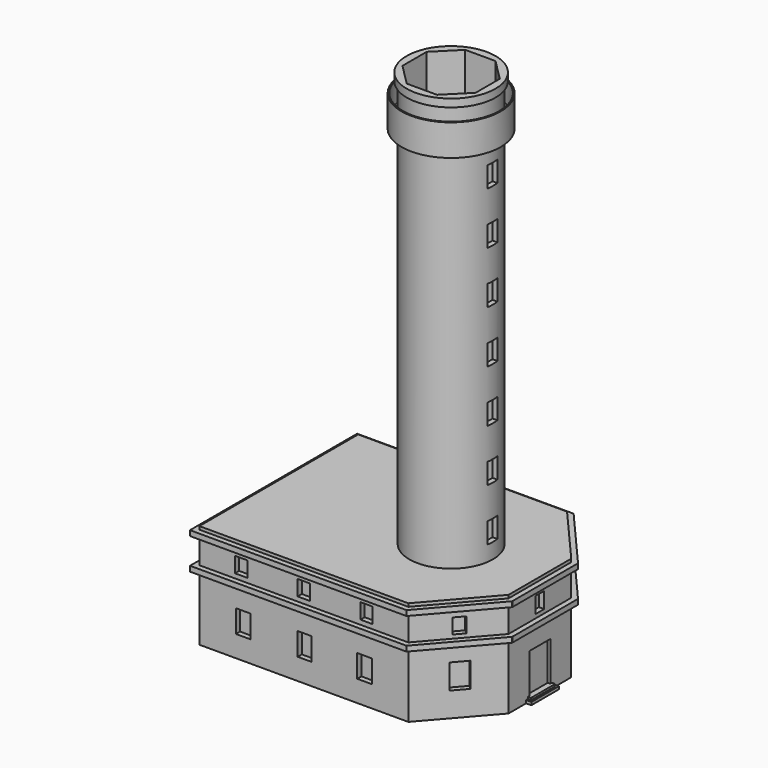
from build123d import *

# Parameters (mm, degrees)
F1_DEPTH  = 50.8
F2_R      = 20.32
F3_DEPTH  = 177.8
F5_DEPTH  = 381
F6_W      = 101.6
F6_H      = 2.54
F7_DEPTH  = 2.54
F8_W      = 38.7089666615
F8_H      = 2.54
F9_DEPTH  = 2.54
F10_DEPTH = 1.143
F11_DEPTH = 1.143
F12_DEPTH = 1.143
F13_DEPTH = 1.143
F14_W     = 38.1
F14_H     = 2.54
F15_DEPTH = 2.54
F16_DEPTH = 0.889
F17_DEPTH = 0.889
F18_W     = 38.7089666615
F18_H     = 2.54
F19_DEPTH = 2.54
F20_W     = 101.6
F20_H     = 2.54
F21_DEPTH = 2.54
F22_DEPTH = 0.889
F23_DEPTH = 0.889
F24_DEPTH = 1.143
F25_DEPTH = 1.143
F27_DEPTH = 2.54
F29_DEPTH = 1.27
F30_DEPTH = 1.524
F31_DEPTH = 2.54
F28_W     = 5.0940667279
F28_H     = 7.758654654
F32_DEPTH = 2.54
F33_R     = 24.13
F33_R_2   = 20.32
F34_DEPTH = 5.08
F35_R     = 20.32
F36_DEPTH = 15.24
F37_R     = 21.59
F37_R_2   = 20.32
F38_DEPTH = 3.81
F39_R     = 24.13
F39_R_2   = 23.495
F40_DEPTH = 10.16
F41_W     = 6.827371195
F41_H     = 9.7158756107
F41_W_2   = 11.0288318247
F41_H_2   = 20.7330156118
F41_W_3   = 6.8273767829
F41_H_3   = 8.1403255463
F41_W_4   = 6.0395970941
F42_DEPTH = 2.54
F43_W     = 7.0659834892
F43_H     = 11.040600948
F43_W_2   = 6.8451717962
F43_W_3   = 5.9624109417
F43_H_2   = 7.5072459877
F43_W_4   = 5.9624111746
F44_DEPTH = 2.54
F45_W     = 9.3363560736
F45_H     = 11.9140176103
F45_W_2   = 5.0487220287
F45_H_2   = 6.8554915488
F46_DEPTH = 2.54
F47_W     = 8.1120701507
F47_H     = 12.0682595298
F47_W_2   = 5.420149304
F47_H_2   = 7.3144324124
F48_DEPTH = 2.54
F49_W     = 5.7560801506
F49_H     = 7.2415210307
F49_W_2   = 8.1699229777
F49_H_2   = 11.5121612325
F49_W_3   = 10.0267203525
F49_H_3   = 19.1327799112
F50_DEPTH = 2.54
F51_W     = 5.8573530426
F51_H     = 10.0520360901
F52_DEPTH = 25.4
F53_W     = 5.1205269992
F53_H     = 8.2716196775
F54_DEPTH = 15.24


with BuildPart() as f1:
    # F0 (on Top) → F1 (new body)
    with BuildSketch(Plane.XY):
        Polygon((-50.8, -48.26), (50.8, -48.26), (76.2, -19.05), (76.2, 19.05), (50.8, 48.26), (-50.8, 48.26), align=None)
    extrude(amount=F1_DEPTH)

    # F2 (on face) → F3 (join)
    with BuildSketch(Plane.XY.offset(50.8)):
        with Locations((33.02, 0)):
            Circle(F2_R)
    extrude(amount=F3_DEPTH)

    # F4 (on Top) → F5 (cut)
    with BuildSketch(Plane.XY):
        Polygon((50.8, 0), (50.8, 7.364717139), (40.384717139, 17.78), (25.655282861, 17.78), (15.24, 7.364717139), (15.24, -7.364717139), (25.655282861, -17.78), (40.384717139, -17.78), (50.8, -7.364717139), align=None)
    extrude(amount=F5_DEPTH, mode=Mode.SUBTRACT)

    # F6 (on face) → F7 (join)
    with BuildSketch(Plane(origin=(0, 48.26, 0), x_dir=(-1, 0, 0), z_dir=(0, 1, 0))):
        with Locations((0, 48.006)):
            Rectangle(F6_W, F6_H)
        with Locations((0, 32.766)):
            Rectangle(F6_W, F6_H)
    extrude(amount=F7_DEPTH)

    # F8 (on face) → F9 (join)
    with BuildSketch(Plane(origin=(52.8232508073, 45.9332615716, 0), x_dir=(-0.6561787149, 0.7546055222, 0), z_dir=(0.7546055222, 0.6561787149, 0))):
        with Locations((-16.2710995493, 48.006)):
            Rectangle(F8_W, F8_H)
        with Locations((-16.2710995493, 32.766)):
            Rectangle(F8_W, F8_H)
    extrude(amount=F9_DEPTH)

    # F10 (add): a face of the model
    f10_faces = [f1.faces().sort_by_distance(p)[0] for p in [
        (50.8, 49.53, 48.006),
    ]]
    extrude(f10_faces, amount=F10_DEPTH)

    # F11 (add): a face of the model
    f11_faces = [f1.faces().sort_by_distance(p)[0] for p in [
        (52.3298490131, 49.5903034897, 48.006),
    ]]
    extrude(f11_faces, amount=F11_DEPTH)

    # F12 (add): a face of the model
    f12_faces = [f1.faces().sort_by_distance(p)[0] for p in [
        (50.8, 49.53, 32.766),
    ]]
    extrude(f12_faces, amount=F12_DEPTH)

    # F13 (add): a face of the model
    f13_faces = [f1.faces().sort_by_distance(p)[0] for p in [
        (52.3298490131, 49.5903034897, 32.766),
    ]]
    extrude(f13_faces, amount=F13_DEPTH)

    # F14 (on face) → F15 (join)
    with BuildSketch(Plane.YZ.offset(76.2)):
        with Locations((0, 48.006)):
            Rectangle(F14_W, F14_H)
        with Locations((0, 32.766)):
            Rectangle(F14_W, F14_H)
    extrude(amount=F15_DEPTH)

    # F16 (add): faces of the model
    f16_faces = [f1.faces().sort_by_distance(p)[0] for p in [
        (77.47, 19.05, 48.006),
        (77.47, 19.05, 32.766),
    ]]
    extrude(f16_faces, amount=F16_DEPTH)

    # F17 (add): faces of the model
    f17_faces = [f1.faces().sort_by_distance(p)[0] for p in [
        (77.6695240131, 20.327846968, 48.006),
        (77.6695240131, 20.327846968, 32.766),
    ]]
    extrude(f17_faces, amount=F17_DEPTH)

    # F18 (on face) → F19 (join)
    with BuildSketch(Plane(origin=(52.8232508073, -45.9332615716, 0), x_dir=(0.6561787149, 0.7546055222, 0), z_dir=(0.7546055222, -0.6561787149, 0))):
        with Locations((16.2710995493, 48.006)):
            Rectangle(F18_W, F18_H)
        with Locations((16.2710995493, 32.766)):
            Rectangle(F18_W, F18_H)
    extrude(amount=F19_DEPTH)

    # F20 (on face) → F21 (join)
    with BuildSketch(Plane.XZ.offset(48.26)):
        with Locations((0, 48.006)):
            Rectangle(F20_W, F20_H)
        with Locations((0, 32.766)):
            Rectangle(F20_W, F20_H)
    extrude(amount=F21_DEPTH)

    # F22 (add): faces of the model
    f22_faces = [f1.faces().sort_by_distance(p)[0] for p in [
        (77.47, -19.05, 48.006),
        (77.47, -19.05, 32.766),
    ]]
    extrude(f22_faces, amount=F22_DEPTH)

    # F23 (add): faces of the model
    f23_faces = [f1.faces().sort_by_distance(p)[0] for p in [
        (77.6695240131, -20.327846968, 48.006),
        (77.6695240131, -20.327846968, 32.766),
    ]]
    extrude(f23_faces, amount=F23_DEPTH)

    # F24 (add): faces of the model
    f24_faces = [f1.faces().sort_by_distance(p)[0] for p in [
        (51.7583490131, -49.093346968, 48.006),
        (51.7583490131, -49.093346968, 32.766),
    ]]
    extrude(f24_faces, amount=F24_DEPTH)

    # F25 (add): faces of the model
    f25_faces = [f1.faces().sort_by_distance(p)[0] for p in [
        (50.8, -50.2873493477, 48.006),
        (50.8, -50.2873493477, 32.766),
    ]]
    extrude(f25_faces, amount=F25_DEPTH)

    # F26 (on face) → F27 (join)
    with BuildSketch(Plane(origin=(-50.8, 0, 0), x_dir=(0, -1, 0), z_dir=(-1, 0, 0))):
        Polygon((-48.26, 49.276), (-50.8, 49.276), (-50.8, 46.736), (-48.26, 46.736), (48.26, 46.736), (50.8, 46.736), (50.8, 49.276), (48.26, 49.276), align=None)
        Polygon((48.26, 34.036), (-48.26, 34.036), (-50.8, 34.036), (-50.8, 31.496), (-48.26, 31.496), (48.26, 31.496), (50.8, 31.496), (50.8, 34.036), align=None)
    extrude(amount=F27_DEPTH)

    # F28 (on face) → F29 (cut)
    with BuildSketch(Plane.YZ.offset(76.2)):
        Polygon((-6.35, 21.59), (-6.35, 2.4007817265), (6.35, 2.4007817265), (6.35, 21.59), (0, 21.59), align=None)
    extrude(amount=-F29_DEPTH, mode=Mode.SUBTRACT)

    # F28 (on face) → F30 (join)
    with BuildSketch(Plane.YZ.offset(76.2)):
        Polygon((-7.366, 2.4007817265), (-7.366, 1.3964880491), (-6.35, 1.3964880491), (6.35, 1.3964880491), (7.366, 1.3964880491), (7.366, 2.4007817265), (6.35, 2.4007817265), (-6.35, 2.4007817265), align=None)
    extrude(amount=F30_DEPTH)

    # F28 (on face) → F31 (join)
    with BuildSketch(Plane.YZ.offset(76.2)):
        Polygon((-8.382, 0), (0, 0), (6.35, 0), (8.382, 0), (8.382, 1.3964880491), (7.366, 1.3964880491), (6.35, 1.3964880491), (-6.35, 1.3964880491), (-7.366, 1.3964880491), (-8.382, 1.3964880491), align=None)
    extrude(amount=F31_DEPTH)

    # F28 (on face) → F32 (cut)
    with BuildSketch(Plane.YZ.offset(76.2)):
        with Locations((0.0010598451, 39.7888198495)):
            Rectangle(F28_W, F28_H)
    extrude(amount=-F32_DEPTH, mode=Mode.SUBTRACT)

    # F33 (on face) → F34 (join)
    with BuildSketch(Plane.XY.offset(228.6)):
        with Locations((33.02, 0)):
            Circle(F33_R)
        with Locations((33.02, 0)):
            Circle(F33_R_2, mode=Mode.SUBTRACT)
        with Locations((33.02, 0)):
            Circle(F33_R_2)
        Polygon((40.384717139, 17.78), (50.8, 7.364717139), (50.8, -7.364717139), (40.384717139, -17.78), (25.655282861, -17.78), (15.24, -7.364717139), (15.24, 7.364717139), (25.655282861, 17.78), align=None, mode=Mode.SUBTRACT)
    extrude(amount=F34_DEPTH)

    # F39 (on face) → F40 (join)
    with BuildSketch(Plane.XY.offset(233.68)):
        with Locations((33.02, 0)):
            Circle(F39_R)
        with Locations((33.02, 0)):
            Circle(F39_R_2, mode=Mode.SUBTRACT)
    extrude(amount=F40_DEPTH)

    # F41 (on face) → F42 (cut)
    with BuildSketch(Plane(origin=(0, 48.26, 0), x_dir=(-1, 0, 0), z_dir=(0, 1, 0))):
        with Locations((-34.0784108266, 19.2887661979)):
            Rectangle(F41_W, F41_H)
        with Locations((-7.2941081598, 19.2887661979)):
            Rectangle(F41_W, F41_H)
        with Locations((29.7312485054, 10.3665078059)):
            Rectangle(F41_W_2, F41_H_2)
        with Locations((27.8931111097, 39.7708788514)):
            Rectangle(F41_W_3, F41_H_3)
        with Locations((-7.4254050851, 40.0334708393)):
            Rectangle(F41_W_4, F41_H_3)
        with Locations((-33.9471139014, 40.0334708393)):
            Rectangle(F41_W_4, F41_H_3)
    extrude(amount=-F42_DEPTH, mode=Mode.SUBTRACT)

    # F43 (on face) → F44 (cut)
    with BuildSketch(Plane.XZ.offset(48.26)):
        with Locations((-29.5082172379, 15.9119707532)):
            Rectangle(F43_W, F43_H)
        with Locations((0.4118072102, 15.9119707532)):
            Rectangle(F43_W_2, F43_H)
        with Locations((29.5082172379, 15.9119707532)):
            Rectangle(F43_W, F43_H)
        with Locations((30.5021060631, 39.9816092104)):
            Rectangle(F43_W_3, F43_H_2)
        with Locations((-0.0275586499, 39.9865973741)):
            Rectangle(F43_W_4, F43_H_2)
        with Locations((-30.5021060631, 39.9816092104)):
            Rectangle(F43_W_3, F43_H_2)
    extrude(amount=-F44_DEPTH, mode=Mode.SUBTRACT)

    # F45 (on face) → F46 (cut)
    with BuildSketch(Plane(origin=(52.8232508073, 45.9332615716, 0), x_dir=(-0.6561787149, 0.7546055222, 0), z_dir=(0.7546055222, 0.6561787149, 0))):
        with Locations((-15.2770597488, 18.6095112003)):
            Rectangle(F45_W, F45_H)
        with Locations((-15.4854785651, 40.2636621147)):
            Rectangle(F45_W_2, F45_H_2)
    extrude(amount=-F46_DEPTH, mode=Mode.SUBTRACT)

    # F47 (on face) → F48 (cut)
    with BuildSketch(Plane(origin=(52.8232508073, -45.9332615716, 0), x_dir=(0.6561787149, 0.7546055222, 0), z_dir=(0.7546055222, -0.6561787149, 0))):
        with Locations((16.8952397071, 17.9421999492)):
            Rectangle(F47_W, F47_H)
        with Locations((16.6423316114, 39.4750740379)):
            Rectangle(F47_W_2, F47_H_2)
    extrude(amount=-F48_DEPTH, mode=Mode.SUBTRACT)

    # F49 (on face) → F50 (cut)
    with BuildSketch(Plane(origin=(-50.8, 0, 0), x_dir=(0, -1, 0), z_dir=(-1, 0, 0))):
        with Locations((-20.8684261888, 40.021782741)):
            Rectangle(F49_W, F49_H)
        with Locations((20.8684261888, 40.021782741)):
            Rectangle(F49_W, F49_H)
        with Locations((-35.4443062097, 17.4616607837)):
            Rectangle(F49_W_2, F49_H_2)
        with Locations((0.0205757096, 9.5663899556)):
            Rectangle(F49_W_3, F49_H_3)
        with Locations((35.4443062097, 17.4616607837)):
            Rectangle(F49_W_2, F49_H_2)
    extrude(amount=-F50_DEPTH, mode=Mode.SUBTRACT)

    # F51 (on face) → F52 (cut)
    with BuildSketch(Plane.YZ.offset(76.2)):
        with Locations((0, 88.7092192439)):
            Rectangle(F51_W, F51_H)
        with Locations((0, 63.3092192439)):
            Rectangle(F51_W, F51_H)
        with Locations((0, 114.1092192439)):
            Rectangle(F51_W, F51_H)
        with Locations((0, 139.5092192439)):
            Rectangle(F51_W, F51_H)
        with Locations((0, 164.9092192439)):
            Rectangle(F51_W, F51_H)
        with Locations((0, 190.3092192439)):
            Rectangle(F51_W, F51_H)
        with Locations((0, 215.7092192439)):
            Rectangle(F51_W, F51_H)
    extrude(amount=-F52_DEPTH, mode=Mode.SUBTRACT)

    # F53 (on Right) → F54 (cut)
    with BuildSketch(Plane.YZ):
        with Locations((0.0553554855, 54.9743659794)):
            Rectangle(F53_W, F53_H)
    extrude(amount=F54_DEPTH, mode=Mode.SUBTRACT)


with BuildPart() as f36:
    # F35 (on face) → F36 (new body)
    with BuildSketch(Plane.XY.offset(233.68)):
        with Locations((33.02, 0)):
            Circle(F35_R)
        Polygon((15.24, -7.364717139), (15.24, 7.364717139), (25.655282861, 17.78), (40.384717139, 17.78), (50.8, 7.364717139), (50.8, -7.364717139), (40.384717139, -17.78), (25.655282861, -17.78), align=None, mode=Mode.SUBTRACT)
    extrude(amount=F36_DEPTH)

    # F37 (on face) → F38 (join)
    with BuildSketch(Plane.XY.offset(248.92)):
        with Locations((33.02, 0)):
            Circle(F37_R)
        with Locations((33.02, 0)):
            Circle(F37_R_2, mode=Mode.SUBTRACT)
        with Locations((33.02, 0)):
            Circle(F37_R_2)
        Polygon((40.384717139, -17.78), (25.655282861, -17.78), (15.24, -7.364717139), (15.24, 7.364717139), (25.655282861, 17.78), (40.384717139, 17.78), (50.8, 7.364717139), (50.8, -7.364717139), align=None, mode=Mode.SUBTRACT)
    extrude(amount=F38_DEPTH)


solid = Compound([f1.part, f36.part])
